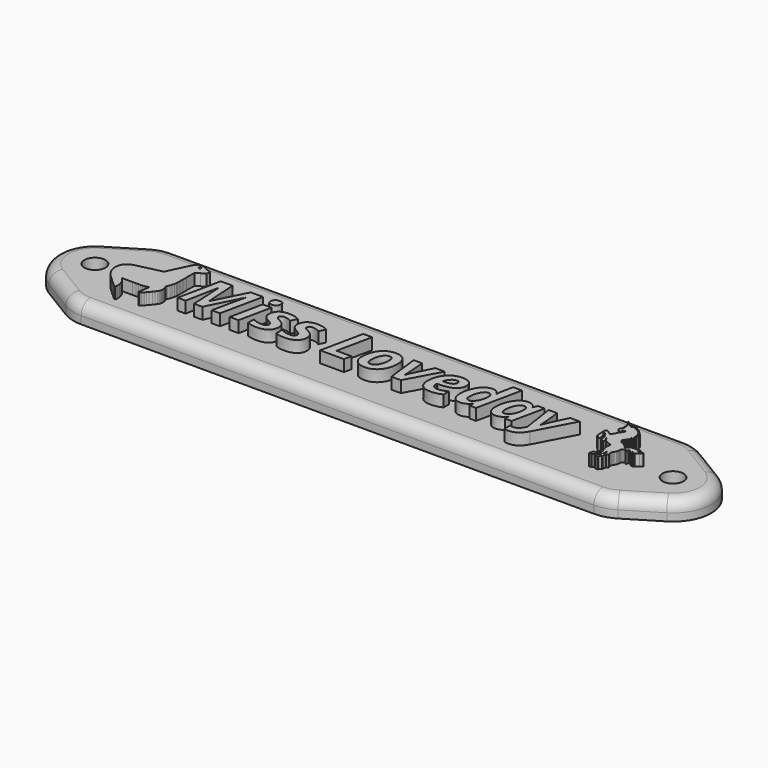
from build123d import *

# Parameters (mm, degrees)
F0_W         = 140
F0_H         = 30.4531101137
F1_DEPTH     = 5
F2_R         = 10
F3_R         = 10
F4_TEXT_SIZE = 15.6755168022
F5_DEPTH     = 3
F7_D         = 5.5
F8_R         = 0.282704
F9_DEPTH     = 3
F11_DEPTH    = 3
F12_R        = 3


# Not quite as in the source:
# - Text() gives the source's letters only with a copy of the font that has no kerning and outlines rounded to 1/6400 em; it was checked with that copy


with BuildPart() as f1:
    # F0 (on Top) → F1 (new body)
    with BuildSketch(Plane.XY):
        Rectangle(F0_W, F0_H)
        Polygon((-95, 0), (-70, -15.2265550569), (-70, 15.2265550569), align=None)
        Polygon((70, 15.2265550569), (70, -15.2265550569), (95, 0), align=None)
    extrude(amount=F1_DEPTH)

    # F2
    f2_edges = [f1.edges().sort_by_distance(p)[0] for p in [
        (-95, 0, 2.5),
        (95, 0, 2.5),
    ]]
    fillet(f2_edges, radius=F2_R)

    # F3
    f3_edges = [f1.edges().sort_by_distance(p)[0] for p in [
        (70, -15.226555, 2.5),
        (-70, -15.226555, 2.5),
        (-70, 15.226555, 2.5),
        (70, 15.226555, 2.5),
    ]]
    fillet(f3_edges, radius=F3_R)

    # F4 (on face) → F5 (join)
    with BuildSketch(Plane.XY.offset(5)):
        with Locations((-50, -5.6431860488)):
            Text('Miss Loveday', F4_TEXT_SIZE, font='Open Sans', font_style=FontStyle.BOLDITALIC, text_align=(TextAlign.LEFT, TextAlign.BOTTOM))
    extrude(amount=F5_DEPTH)

    # F7 (through all)
    with Locations(Plane.XY.offset(5)):
        with Locations((75.7757134551, 0), (-75.7757134551, 0)):
            Hole(F7_D / 2)

    # F8 (on face) → F9 (join)
    with BuildSketch(Plane.XY.offset(5)):
        Polygon((-65.1555724097, -7.7435036488), (-64.4543324097, -8.3903836488), (-63.8004924097, -8.9847836488), (-63.3014124097, -9.4225036488), (-62.9708524097, -9.6913836488), (-62.8232924097, -9.7795036488), (-62.7180524097, -9.7196236488), (-62.6414524097, -9.5731036488), (-62.5945724097, -9.3429036488), (-62.5787324097, -9.0325436488), (-62.6422924097, -8.3105436488), (-62.8250124097, -7.6104636488), (-63.1164524097, -6.9641836488), (-63.5049724097, -6.4027836488), (-63.8716924097, -5.9724636488), (-61.1974124097, -5.9719836488), (-60.2803324097, -5.9702636488), (-59.5541724097, -5.9641836488), (-58.9880124097, -5.9516236488), (-58.5498524097, -5.9301036488), (-58.2078524097, -5.8975436488), (-57.9307324097, -5.8519836488), (-57.6867724097, -5.7909836488), (-57.4439324097, -5.7126636488), (-57.2961724097, -5.6636236488), (-57.1685724097, -5.6267036488), (-57.0750124097, -5.6049836488), (-57.0287724097, -5.6023836488), (-57.0309724097, -5.7204636488), (-57.0682924097, -6.0279836488), (-57.1347324097, -6.4782636488), (-57.2236924097, -7.0245036488), (-57.3161324097, -7.5752636488), (-57.3918524097, -8.0383836488), (-57.4430524097, -8.3649836488), (-57.4619724097, -8.5067036488), (-57.4274524097, -8.6149836488), (-57.3402124097, -8.7239436488), (-57.2267324097, -8.8077036488), (-57.1134524097, -8.8413436488), (-57.0650524097, -8.8237836488), (-56.9908524097, -8.7684236488), (-56.8868924097, -8.6705436488), (-56.7486124097, -8.5251836488), (-56.5720124097, -8.3274636488), (-56.3524124097, -8.0729036488), (-56.0854524097, -7.7567036488), (-55.7666924097, -7.3743436488), (-55.2898924097, -6.7946636488), (-54.9224524097, -6.3341836488), (-54.6503324097, -5.9682636488), (-54.4593324097, -5.6722636488), (-54.3354524097, -5.4220636488), (-54.2646924097, -5.1931036488), (-54.2330124097, -4.9611036488), (-54.2260524097, -4.7016236488), (-54.2434524097, -4.3704636488), (-54.2978924097, -4.0781036488), (-54.3979324097, -3.7933836488), (-54.5517724097, -3.4861036488), (-54.5795724097, -3.4335436488), (-54.5974124097, -3.3871036488), (-54.6041324097, -3.3402636488), (-54.5982124097, -3.2871036488), (-54.5782924097, -3.2206636488), (-54.5431324097, -3.1349436488), (-54.4912924097, -3.0236236488), (-54.4211724097, -2.8803836488), (-54.2238924097, -2.4136236488), (-54.0481324097, -1.8749836488), (-53.9085724097, -1.3157036488), (-53.8202124097, -0.7879436488), (-53.7970124097, -0.3858236488), (-53.7783324097, 0.3344563512), (-53.7664524097, 1.2940563512), (-53.7618924097, 2.4142963512), (-53.7618924097, 5.1182563512), (-52.7145724097, 5.7410563512), (-51.6670524097, 6.3638563512), (-51.5784924097, 6.6506563512), (-51.4904124097, 6.9626563512), (-51.4482924097, 7.1830563512), (-51.4504524097, 7.3322563512), (-51.4949324097, 7.4282563512), (-51.5828524097, 7.4782563512), (-51.7638524097, 7.5458563512), (-52.0116924097, 7.6226563512), (-52.2998524097, 7.6994563512), (-52.8927324097, 7.8718563512), (-53.1930524097, 8.0278563512), (-53.5574524097, 8.2766563512), (-53.9817324097, 8.4458563512), (-54.4176924097, 8.5214563512), (-54.8158924097, 8.4890563512), (-55.1251724097, 8.3802563512), (-55.4367724097, 8.2134563512), (-55.7232124097, 8.0058563512), (-55.9565724097, 7.7746563512), (-56.0316124097, 7.6666563512), (-56.1398924097, 7.4810563512), (-56.2824924097, 7.2146563512), (-56.4614924097, 6.8650563512), (-56.6783324097, 6.4282563512), (-56.9344124097, 5.9018563512), (-57.2314924097, 5.2826563512), (-57.5708924097, 4.5666563512), (-58.9584924097, 1.6295363512), (-62.2777324097, 0.8522163512), (-62.9506924097, 0.6942163512), (-63.5902124097, 0.5427763512), (-64.1817724097, 0.4017363512), (-64.7100124097, 0.2745763512), (-65.1604924097, 0.1651763512), (-65.5184124097, 0.0766163512), (-65.7686124097, 0.0130563512), (-65.8964524097, -0.0225436488), (-66.6711724097, -0.3808236488), (-67.2807324097, -0.8839036488), (-67.7200124097, -1.5086636488), (-67.9834524097, -2.2315436488), (-68.0661324097, -3.0292636488), (-67.9624124097, -3.8786636488), (-67.6670524097, -4.7565036488), (-67.1748524097, -5.6395036488), (-67.0285724097, -5.8496236488), (-66.8744924097, -6.0496636488), (-66.6891724097, -6.2636636488), (-66.4484924097, -6.5158236488), (-66.1286124097, -6.8305036488), (-65.7056924097, -7.2315436488), align=None)
        with Locations((-54.2613854097, 7.5656233512)):
            Circle(F8_R, mode=Mode.SUBTRACT)
    extrude(amount=F9_DEPTH)

    # F10 (on face) → F11 (join)
    with BuildSketch(Plane.XY.offset(5)):
        Polygon((59.2275306848, -6.5195911563), (59.1261026848, -6.8110191563), (59.1469596848, -6.8247341563), (59.1698166848, -6.8364481563), (59.2069596848, -6.8507341563), (59.2478166848, -6.8615911563), (59.3066736848, -6.8713051563), (59.6141026848, -6.8735911563), (59.9246736848, -6.8724481563), (59.9561026848, -6.8524481563), (59.9843876848, -6.8293051563), (60.0101026848, -6.8033051563), (60.0406736848, -6.7650191563), (60.0743876848, -6.7127341563), (60.2169596848, -6.4598771563), (60.2481026848, -6.4221621563), (60.2652446848, -6.4047341563), (60.2929596848, -6.3813051563), (60.3095306848, -6.3984481563), (60.3252446848, -6.4113051563), (60.3395306848, -6.4204481563), (60.3466736848, -6.4235911563), (60.3532446848, -6.4258771563), (60.3598166848, -6.4273051563), (60.3661026848, -6.4281621563), (60.3723876848, -6.4281621563), (60.3783876848, -6.4275911563), (60.3841026848, -6.4264481563), (60.3898166848, -6.4244481563), (60.4009596848, -6.4195911563), (60.4115306848, -6.4127341563), (60.4266736848, -6.4001621563), (60.4818166848, -6.3495911563), (60.4923876848, -6.3427341563), (60.5035306848, -6.3378771563), (60.5092446848, -6.3361621563), (60.5149596848, -6.3347341563), (60.5209596848, -6.3341621563), (60.5272446848, -6.3341621563), (60.5335306848, -6.3350191563), (60.5401026848, -6.3364481563), (60.5466736848, -6.3387341563), (60.5535306848, -6.3418771563), (60.5681026848, -6.3510191563), (60.5835306848, -6.3638771563), (60.6001026848, -6.3813051563), (60.6026736848, -6.3321621563), (60.6095306848, -6.2873051563), (60.6201026848, -6.2464481563), (60.6386736848, -6.1961621563), (60.6672446848, -6.1387341563), (60.7521026848, -5.9827341563), (60.7709596848, -5.9327341563), (60.7815306848, -5.8918771563), (60.7886736848, -5.8473051563), (60.7915306848, -5.7984481563), (60.7903876848, -5.7633051563), (60.7843876848, -5.7055911563), (60.8186736848, -5.6941621563), (60.8503876848, -5.6793051563), (60.8803876848, -5.6610191563), (60.9083876848, -5.6401621563), (60.9438166848, -5.6084481563), (61.0766736848, -5.4427341563), (61.2143876848, -5.2755911563), (61.2192446848, -5.2715911563), (61.2246736848, -5.2678771563), (61.2338166848, -5.2627341563), (61.2478166848, -5.2570191563), (61.2715306848, -5.2501621563), (61.3755306848, -5.2258771563), (61.3881026848, -5.2207341563), (61.3938166848, -5.2175911563), (61.3986736848, -5.2141621563), (61.4606736848, -5.1553051563), (61.5215306848, -5.0913051563), (61.5726736848, -5.0298771563), (61.6121026848, -4.9693051563), (61.6409596848, -4.9095911563), (61.6603876848, -4.8501621563), (61.6721026848, -4.7913051563), (61.6769596848, -4.7324481563), (61.6752446848, -4.6538771563), (61.6269596848, -4.1904481563), (61.6321026848, -4.1201621563), (61.6443876848, -4.0473051563), (61.7003876848, -4.1458771563), (61.7478166848, -4.2533051563), (61.7858166848, -4.3701621563), (61.8138166848, -4.4970191563), (61.8309596848, -4.6344481563), (61.8366736848, -4.7835911563), (61.8286736848, -4.9684481563), (61.7061026848, -5.0818771563), (61.5386736848, -5.2684481563), (61.2452446848, -5.6430191563), (60.9072446848, -6.0127341563), (60.9198166848, -6.0990191563), (60.9229596848, -6.1758771563), (60.9183876848, -6.2447341563), (60.9072446848, -6.3075911563), (60.8869596848, -6.3793051563), (60.7981026848, -6.6404481563), (60.7875306848, -6.7035911563), (60.7838166848, -6.7553051563), (60.7843876848, -6.8110191563), (60.8012446848, -6.8238771563), (60.8195306848, -6.8350191563), (60.8395306848, -6.8444481563), (60.8721026848, -6.8561621563), (60.9078166848, -6.8647341563), (60.9592446848, -6.8724481563), (61.2086736848, -6.8733051563), (61.4601026848, -6.8724481563), (61.4638166848, -6.8615911563), (61.4683876848, -6.8515911563), (61.4726736848, -6.8444481563), (61.4772446848, -6.8381621563), (61.4826736848, -6.8324481563), (61.4886736848, -6.8273051563), (61.4949596848, -6.8227341563), (61.5021026848, -6.8190191563), (61.5101026848, -6.8155911563), (61.5183876848, -6.8130191563), (61.5306736848, -6.8104481563), (61.5441026848, -6.8090191563), (61.5623876848, -6.8090191563), (61.5829596848, -6.8110191563), (61.5955306848, -6.7573051563), (61.6135306848, -6.7093051563), (61.6366736848, -6.6658771563), (61.6635306848, -6.6264481563), (61.7043876848, -6.5787341563), (61.9272446848, -6.3595911563), (61.9543876848, -6.3201621563), (61.9772446848, -6.2767341563), (61.9955306848, -6.2287341563), (62.0043876848, -6.1935911563), (62.0129596848, -6.1355911563), (62.1969596848, -6.1355911563), (62.1995306848, -5.9915911563), (62.2275306848, -5.7481621563), (62.2661026848, -5.4318771563), (62.2689596848, -5.3093051563), (62.2583876848, -5.1527341563), (62.2926736848, -5.1133051563), (62.3401026848, -5.0684481563), (62.4126736848, -5.0121621563), (62.6481026848, -4.8421621563), (62.6943876848, -4.7964481563), (62.7198166848, -4.7664481563), (62.7498166848, -4.7230191563), (62.7483876848, -4.6904481563), (62.7435306848, -4.6584481563), (62.7332446848, -4.6155911563), (62.7146736848, -4.5621621563), (62.5821026848, -4.2530191563), (62.5732446848, -4.2178771563), (62.5655306848, -4.1701621563), (62.5589596848, -4.0493051563), (62.5638166848, -3.9367341563), (62.5786736848, -3.8324481563), (62.6021026848, -3.7353051563), (62.6412446848, -3.6230191563), (62.6986736848, -3.5010191563), (62.8169596848, -3.3067341563), (62.9341026848, -3.1258771563), (63.1298166848, -2.7533051563), (63.2312446848, -2.5078771563), (63.2715306848, -2.3861621563), (63.3026736848, -2.2661621563), (63.3198166848, -2.1653051563), (63.3315306848, -2.0133051563), (63.3415306848, -1.6253051563), (63.3492446848, -1.5790191563), (63.3543876848, -1.5581621563), (63.3641026848, -1.5290191563), (63.3886736848, -1.4750191563), (63.4286736848, -1.4064481563), (63.4758166848, -1.3413051563), (63.5432446848, -1.2653051563), (63.6181026848, -1.1953051563), (63.7155306848, -1.1195911563), (63.8346736848, -1.0427341563), (63.9715306848, -0.9701621563), (64.1009596848, -0.9150191563), (64.1463876848, -0.9321621563), (64.1872446848, -0.9541621563), (64.2238166848, -0.9798771563), (64.2569596848, -1.0095911563), (64.2869596848, -1.0424481563), (64.3223876848, -1.0904481563), (64.3609596848, -1.1561621563), (64.4263876848, -1.2995911563), (64.4758166848, -1.4173051563), (64.5309596848, -1.5290191563), (64.5538166848, -1.4598771563), (64.5803876848, -1.3390191563), (64.6495306848, -0.9473051563), (64.6721026848, -0.8778771563), (64.6889596848, -0.8393051563), (64.7152446848, -0.7921621563), (65.1452446848, -0.7921621563), (65.2666736848, -0.9138771563), (65.6092446848, -1.2344481563), (65.6501026848, -1.2821621563), (65.6978166848, -1.3447341563), (65.7478166848, -1.3498771563), (66.1275306848, -1.4144481563), (66.1883876848, -1.4138771563), (66.2306736848, -1.4081621563), (66.2569596848, -1.4013051563), (66.2812446848, -1.3918771563), (66.3035306848, -1.3795911563), (66.3238166848, -1.3644481563), (66.3415306848, -1.3458771563), (66.3563876848, -1.3235911563), (66.3629596848, -1.3113051563), (66.3735306848, -1.2833051563), (66.2275306848, -1.2821621563), (66.1441026848, -1.2733051563), (66.0823876848, -1.2613051563), (66.0261026848, -1.2438771563), (65.9875306848, -1.2273051563), (65.9523876848, -1.2070191563), (65.9309596848, -1.1915911563), (65.9112446848, -1.1744481563), (65.8932446848, -1.1555911563), (65.8772446848, -1.1350191563), (65.8629596848, -1.1124481563), (65.8506736848, -1.0878771563), (65.8403876848, -1.0613051563), (65.8321026848, -1.0327341563), (65.8238166848, -0.9855911563), (65.8212446848, -0.9513051563), (65.8206736848, -0.9150191563), (65.8769596848, -0.9215911563), (65.9286736848, -0.9324481563), (65.9921026848, -0.9524481563), (66.0501026848, -0.9781621563), (66.1301026848, -1.0233051563), (66.3486736848, -1.1595911563), (66.4066736848, -1.1853051563), (66.4695306848, -1.2058771563), (66.5035306848, -1.2135911563), (66.5578166848, -1.2218771563), (66.5652446848, -1.2207341563), (66.5718166848, -1.2190191563), (66.5781026848, -1.2164481563), (66.5838166848, -1.2135911563), (66.5892446848, -1.2104481563), (66.5941026848, -1.2064481563), (66.5983876848, -1.2024481563), (66.6023876848, -1.1978771563), (66.6092446848, -1.1875911563), (66.6149596848, -1.1758771563), (66.6195306848, -1.1633051563), (66.6246736848, -1.1427341563), (66.6441026848, -1.0330191563), (66.6486736848, -1.0204481563), (66.6543876848, -1.0090191563), (66.6615306848, -0.9987341563), (66.6655306848, -0.9944481563), (66.6698166848, -0.9901621563), (66.6746736848, -0.9864481563), (66.6801026848, -0.9833051563), (66.6861026848, -0.9804481563), (66.6923876848, -0.9781621563), (66.6992446848, -0.9764481563), (66.7143876848, -0.9744481563), (66.7229596848, -0.9744481563), (66.7421026848, -0.9764481563), (67.4178166848, -0.5464481563), (67.8358166848, -0.3101621563), (67.8895306848, -0.2658771563), (67.9255306848, -0.2293051563), (67.9578166848, -0.1895911563), (67.9849596848, -0.1464481563), (68.0069596848, -0.0995911563), (68.0181026848, -0.0661621563), (68.0266736848, -0.0310191563), (68.0318166848, 0.0064088437), (67.9761026848, 0.0318378437), (67.9172446848, 0.0512658437), (67.8558166848, 0.0652658437), (67.7595306848, 0.0766948437), (67.6249596848, 0.0784088437), (67.3783876848, 0.0549808437), (66.8869596848, -0.0018771563), (66.7578166848, 0.0009808437), (66.6669596848, 0.0138378437), (66.6098166848, 0.0289808437), (66.5555306848, 0.0492658437), (66.5046736848, 0.0761228437), (66.4803876848, 0.0921228437), (66.4349596848, 0.1292658437), (66.4572446848, 0.1621228437), (66.4823876848, 0.1924088437), (66.5192446848, 0.2292658437), (66.5701026848, 0.2704088437), (66.8421026848, 0.4592658437), (66.8789596848, 0.4958378437), (66.9041026848, 0.5261228437), (66.9263876848, 0.5592658437), (66.6349596848, 0.5212658437), (66.2906736848, 0.5109808437), (64.8941026848, 0.5749808437), (64.7203876848, 0.5506948437), (64.5975306848, 0.5192658437), (64.5192446848, 0.4909808437), (64.4081026848, 0.4364088437), (64.2852446848, 0.3569808437), (64.1538166848, 0.2541228437), (63.5326736848, -0.3198771563), (63.4635306848, -0.3661621563), (63.3641026848, -0.4235911563), (63.3063876848, -0.2847341563), (63.2363876848, -0.1581621563), (63.1552446848, -0.0427341563), (63.0638166848, 0.0624088437), (62.9103876848, 0.2038378437), (62.7406736848, 0.3286948437), (62.4321026848, 0.5115518437), (61.5375306848, 0.9929808437), (61.3669596848, 1.1172658437), (61.2123876848, 1.2575518437), (61.1203876848, 1.3618378437), (61.0381026848, 1.4761228437), (60.9669596848, 1.6015518437), (60.9083876848, 1.7395518437), (60.8841026848, 1.8132658437), (60.8458166848, 1.9718378437), (60.8883876848, 2.0469808437), (60.9089596848, 2.0755518437), (60.9275306848, 2.0966948437), (60.9426736848, 2.1106948437), (60.9595306848, 2.1235518437), (60.9778166848, 2.1346948437), (60.9978166848, 2.1441228437), (61.0198166848, 2.1518378437), (61.0438166848, 2.1569808437), (61.0701026848, 2.1601228437), (61.0989596848, 2.1609808437), (61.1195306848, 2.1598378437), (61.1529596848, 2.1561228437), (61.1612446848, 2.1744088437), (61.1666736848, 2.1924088437), (61.1701026848, 2.2104088437), (61.1712446848, 2.2281228437), (61.1703876848, 2.2455518437), (61.1663876848, 2.2712658437), (61.1598166848, 2.2961228437), (61.1478166848, 2.3272658437), (61.1086736848, 2.4166948437), (61.1066736848, 2.4261228437), (61.1063876848, 2.4306948437), (61.1063876848, 2.4346948437), (61.1069596848, 2.4386948437), (61.1081026848, 2.4424088437), (61.1095306848, 2.4458378437), (61.1118166848, 2.4486948437), (61.1143876848, 2.4515518437), (61.1178166848, 2.4541228437), (61.1218166848, 2.4564088437), (61.1266736848, 2.4584088437), (61.1321026848, 2.4601228437), (61.1381026848, 2.4612658437), (61.1529596848, 2.4632658437), (61.1729596848, 2.4646948437), (61.1909596848, 2.4641228437), (61.2072446848, 2.4621228437), (61.2223876848, 2.4589808437), (61.2409596848, 2.4526948437), (61.2621026848, 2.4432658437), (61.3232446848, 2.4124088437), (61.3418166848, 2.4064088437), (61.3572446848, 2.4032658437), (61.3738166848, 2.4015518437), (61.3858166848, 2.4012658437), (61.3986736848, 2.4018378437), (61.4681026848, 2.6566948437), (61.4861026848, 2.6975518437), (61.5021026848, 2.7255518437), (61.5206736848, 2.7512658437), (61.5346736848, 2.7666948437), (61.5501026848, 2.7809808437), (61.5669596848, 2.7935518437), (61.5855306848, 2.8046948437), (61.6055306848, 2.8138378437), (61.6275306848, 2.8212658437), (61.6515306848, 2.8269808437), (61.6775306848, 2.8304088437), (61.7058166848, 2.8315518437), (61.6746736848, 2.9669808437), (61.6735306848, 2.9815518437), (61.6741026848, 2.9958378437), (61.6835306848, 3.0461228437), (61.7058166848, 3.1386948437), (61.7255306848, 3.1401228437), (61.7438166848, 3.1398378437), (61.7601026848, 3.1378378437), (61.7752446848, 3.1344088437), (61.7935306848, 3.1284088437), (61.8146736848, 3.1186948437), (61.8761026848, 3.0881228437), (61.8946736848, 3.0821228437), (61.9098166848, 3.0789808437), (61.9266736848, 3.0769808437), (61.9386736848, 3.0766948437), (61.9515306848, 3.0772658437), (61.9629596848, 3.1369808437), (61.9675306848, 3.1935518437), (61.9658166848, 3.2475518437), (61.9592446848, 3.2986948437), (61.9446736848, 3.3635518437), (61.9092446848, 3.4681228437), (61.8615306848, 3.6032658437), (61.8529596848, 3.6415518437), (61.8489596848, 3.6789808437), (61.8492446848, 3.7038378437), (61.8523876848, 3.7284088437), (61.8586736848, 3.7529808437), (61.8683876848, 3.7775518437), (61.8746736848, 3.7898378437), (61.8901026848, 3.8144088437), (61.9301026848, 3.8101228437), (61.9761026848, 3.8009808437), (62.0266736848, 3.7852658437), (62.2338166848, 3.7049808437), (62.2703876848, 3.6972658437), (62.3198166848, 3.6915518437), (62.3098166848, 3.8041228437), (62.2903876848, 3.9075518437), (62.2572446848, 4.0218378437), (62.1938166848, 4.1795518437), (62.1001026848, 4.3806948437), (62.0129596848, 4.6126948437), (62.0946736848, 4.6686948437), (62.1215306848, 4.6921228437), (62.1361026848, 4.7084088437), (62.1435306848, 4.7192658437), (62.1489596848, 4.7298378437), (62.1529596848, 4.7404088437), (62.1549596848, 4.7512658437), (62.1558166848, 4.7624088437), (62.1549596848, 4.7741228437), (62.1526736848, 4.7861228437), (62.1472446848, 4.8058378437), (62.1175306848, 4.8784088437), (62.0741026848, 4.9812658437), (62.1566736848, 5.0106948437), (62.2218166848, 5.0412658437), (62.2715306848, 5.0715518437), (62.3075306848, 5.0992658437), (62.3401026848, 5.1306948437), (62.3621026848, 5.1566948437), (62.3815306848, 5.1849808437), (62.3986736848, 5.2158378437), (62.4132446848, 5.2489808437), (62.4252446848, 5.2852658437), (62.4341026848, 5.3241228437), (62.4401026848, 5.3661228437), (62.4426736848, 5.4112658437), (62.1975306848, 5.4118378437), (62.1318166848, 5.4195518437), (62.0912446848, 5.4284088437), (62.0632446848, 5.4369808437), (62.0372446848, 5.4481228437), (62.0138166848, 5.4612658437), (61.9995306848, 5.4715518437), (61.9866736848, 5.4832658437), (61.9746736848, 5.4961228437), (61.9643876848, 5.5101228437), (61.9598166848, 5.5178378437), (61.9515306848, 5.5341228437), (61.9652446848, 5.7164088437), (61.9761026848, 5.8249808437), (61.9752446848, 5.8698378437), (61.9675306848, 5.9355518437), (61.9515306848, 6.0255518437), (62.0106736848, 6.0324088437), (62.0532446848, 6.0415518437), (62.0863876848, 6.0524088437), (62.1118166848, 6.0638378437), (62.1306736848, 6.0746948437), (62.1478166848, 6.0869808437), (62.1632446848, 6.1009808437), (62.1738166848, 6.1124088437), (62.1835306848, 6.1249808437), (62.1892446848, 6.1338378437), (62.1969596848, 6.1484088437), (62.1403876848, 6.1749808437), (62.0638166848, 6.2026948437), (61.9143876848, 6.2415518437), (61.5581026848, 6.3238378437), (61.4818166848, 6.3518378437), (61.4386736848, 6.3715518437), (61.3986736848, 6.3938378437), (61.3915306848, 6.4178378437), (61.3875306848, 6.4412658437), (61.3861026848, 6.4646948437), (61.3866736848, 6.4878378437), (61.3915306848, 6.5221228437), (61.4029596848, 6.5666948437), (61.4641026848, 6.7395518437), (61.4669596848, 6.7578378437), (61.4683876848, 6.7755518437), (61.4672446848, 6.7929808437), (61.4638166848, 6.8098378437), (61.4575306848, 6.8261228437), (61.4481026848, 6.8418378437), (61.4355306848, 6.8566948437), (61.4189596848, 6.8712658437), (61.3986736848, 6.8852658437), (61.3749596848, 6.8666948437), (61.2441026848, 6.7486948437), (61.2258166848, 6.7375518437), (61.2075306848, 6.7289808437), (61.1949596848, 6.7249808437), (61.1826736848, 6.7224088437), (61.1698166848, 6.7218378437), (61.1572446848, 6.7229808437), (61.1443876848, 6.7264088437), (61.1312446848, 6.7315518437), (61.1183876848, 6.7395518437), (61.1049596848, 6.7495518437), (61.0915306848, 6.7624088437), (61.0881026848, 6.8326948437), (61.0786736848, 6.8969808437), (61.0586736848, 6.9801228437), (60.9815306848, 7.2421228437), (60.9721026848, 7.3064088437), (60.9686736848, 7.3766948437), (60.9463876848, 7.3815518437), (60.9269596848, 7.3838378437), (60.9101026848, 7.3838378437), (60.8955306848, 7.3812658437), (60.8889596848, 7.3789808437), (60.8829596848, 7.3764088437), (60.8772446848, 7.3735518437), (60.8721026848, 7.3701228437), (60.8675306848, 7.3661228437), (60.8592446848, 7.3572658437), (60.8521026848, 7.3469808437), (60.8461026848, 7.3358378437), (60.8386736848, 7.3175518437), (60.8129596848, 7.2401228437), (60.8069596848, 7.2289808437), (60.7998166848, 7.2186948437), (60.7915306848, 7.2098378437), (60.7869596848, 7.2058378437), (60.7818166848, 7.2024088437), (60.7763876848, 7.1992658437), (60.7703876848, 7.1966948437), (60.7638166848, 7.1946948437), (60.7569596848, 7.1929808437), (60.7412446848, 7.1915518437), (60.7229596848, 7.1924088437), (60.4975306848, 7.1929808437), (60.4635306848, 7.1984088437), (60.4403876848, 7.2044088437), (60.4192446848, 7.2126948437), (60.4063876848, 7.2195518437), (60.3946736848, 7.2278378437), (60.3843876848, 7.2369808437), (60.3755306848, 7.2478378437), (60.3681026848, 7.2601228437), (60.3621026848, 7.2735518437), (60.3578166848, 7.2889808437), (60.3563876848, 7.2972658437), (60.3543876848, 7.3152658437), (60.3458166848, 7.3412658437), (60.3412446848, 7.3629808437), (60.3401026848, 7.3812658437), (60.3409596848, 7.3889808437), (60.3423876848, 7.3961228437), (60.3446736848, 7.4024088437), (60.3478166848, 7.4081228437), (60.3512446848, 7.4129808437), (60.3555306848, 7.4172658437), (60.3603876848, 7.4212658437), (60.3658166848, 7.4244088437), (60.3715306848, 7.4272658437), (60.3843876848, 7.4315518437), (60.3986736848, 7.4344088437), (60.4301026848, 7.4372658437), (60.4943876848, 7.4418378437), (60.5086736848, 7.4446948437), (60.5218166848, 7.4489808437), (60.5275306848, 7.4518378437), (60.5329596848, 7.4549808437), (60.5378166848, 7.4586948437), (60.5421026848, 7.4629808437), (60.5455306848, 7.4681228437), (60.5486736848, 7.4735518437), (60.5509596848, 7.4801228437), (60.5523876848, 7.4869808437), (60.5532446848, 7.4949808437), (60.5532446848, 7.5035518437), (60.5503876848, 7.5235518437), (60.5475306848, 7.5349808437), (60.5386736848, 7.5609808437), (60.5335306848, 7.5704088437), (60.5272446848, 7.5789808437), (60.5201026848, 7.5864088437), (60.5121026848, 7.5929808437), (60.5029596848, 7.5989808437), (60.4932446848, 7.6038378437), (60.4718166848, 7.6118378437), (60.4475306848, 7.6169808437), (60.4072446848, 7.6209808437), (60.3332446848, 7.6206948437), (60.1669596848, 7.6166948437), (60.1278166848, 7.6215518437), (60.1043876848, 7.6275518437), (60.0835306848, 7.6364088437), (60.0743876848, 7.6418378437), (60.0658166848, 7.6481228437), (60.0583876848, 7.6552658437), (60.0518166848, 7.6635518437), (60.0461026848, 7.6724088437), (60.0415306848, 7.6826948437), (60.0378166848, 7.6938378437), (60.0355306848, 7.7061228437), (60.0341026848, 7.7195518437), (60.0355306848, 7.7504088437), (60.0381026848, 7.7678378437), (60.0475306848, 7.8066948437), (60.0215306848, 7.8081228437), (59.9981026848, 7.8069808437), (59.9769596848, 7.8032658437), (59.9581026848, 7.7978378437), (59.9409596848, 7.7901228437), (59.9255306848, 7.7809808437), (59.9115306848, 7.7706948437), (59.8923876848, 7.7526948437), (59.8641026848, 7.7195518437), (59.8195306848, 7.6661228437), (59.8001026848, 7.6484088437), (59.7861026848, 7.6381228437), (59.7703876848, 7.6292658437), (59.7529596848, 7.6218378437), (59.7338166848, 7.6164088437), (59.7126736848, 7.6132658437), (59.6889596848, 7.6124088437), (59.6623876848, 7.6141228437), (59.6175306848, 7.6224088437), (59.6141026848, 7.6372658437), (59.6092446848, 7.6509808437), (59.6032446848, 7.6635518437), (59.5963876848, 7.6749808437), (59.5858166848, 7.6889808437), (59.5681026848, 7.7081228437), (59.5223876848, 7.7544088437), (59.5118166848, 7.7684088437), (59.5049596848, 7.7801228437), (59.4992446848, 7.7926948437), (59.4946736848, 7.8066948437), (59.4966736848, 7.8412658437), (59.5023876848, 7.8724088437), (59.5115306848, 7.9001228437), (59.5232446848, 7.9252658437), (59.5372446848, 7.9481228437), (59.5583876848, 7.9764088437), (59.6412446848, 8.0775518437), (59.6546736848, 8.1009808437), (59.6658166848, 8.1269808437), (59.6738166848, 8.1555518437), (59.6786736848, 8.1875518437), (59.6798166848, 8.2109808437), (59.6789596848, 8.2364088437), (59.5952446848, 8.2169808437), (59.5186736848, 8.1904088437), (59.4481026848, 8.1578378437), (59.3612446848, 8.1069808437), (59.2621026848, 8.0344088437), (58.9206736848, 7.7566948437), (58.8338166848, 7.7058378437), (58.7632446848, 7.6732658437), (58.6866736848, 7.6466948437), (58.6315306848, 7.6329808437), (58.5732446848, 7.6224088437), (58.5746736848, 7.8961228437), (58.5809596848, 7.9389808437), (58.5883876848, 7.9709808437), (58.5961026848, 7.9926948437), (58.6052446848, 8.0129808437), (58.6163876848, 8.0312658437), (58.6252446848, 8.0421228437), (58.6346736848, 8.0521228437), (58.6061026848, 8.0501228437), (58.5789596848, 8.0449808437), (58.5535306848, 8.0372658437), (58.5295306848, 8.0266948437), (58.5069596848, 8.0141228437), (58.4755306848, 7.9918378437), (58.4466736848, 7.9664088437), (58.4035306848, 7.9204088437), (58.3106736848, 7.8118378437), (58.2978166848, 7.8006948437), (58.2849596848, 7.7918378437), (58.2721026848, 7.7855518437), (58.2658166848, 7.7835518437), (58.2592446848, 7.7824088437), (58.2526736848, 7.7821228437), (58.2461026848, 7.7826948437), (58.2395306848, 7.7841228437), (58.2326736848, 7.7864088437), (58.2258166848, 7.7898378437), (58.2189596848, 7.7944088437), (58.2121026848, 7.7998378437), (58.2049596848, 7.8066948437), (58.1581026848, 7.8489808437), (58.1015306848, 7.8906948437), (58.0046736848, 7.9486948437), (57.8758166848, 8.0221228437), (57.8581026848, 8.0346948437), (57.8363876848, 8.0521228437), (57.6346736848, 8.2529808437), (57.2026736848, 8.7398378437), (56.8535306848, 9.0964088437), (56.8435306848, 9.1029808437), (56.8046736848, 9.1244088437), (56.7452446848, 9.1506948437), (56.7009596848, 9.1655518437), (56.6766736848, 9.1712658437), (56.6595306848, 9.1735518437), (56.6441026848, 9.1738378437), (56.6346736848, 9.1729808437), (56.6263876848, 9.1709808437), (56.6226736848, 9.1695518437), (56.6189596848, 9.1678378437), (56.6158166848, 9.1658378437), (56.6129596848, 9.1635518437), (56.6103876848, 9.1606948437), (56.6081026848, 9.1578378437), (57.2415306848, 8.2866948437), (57.8363876848, 7.3766948437), (57.8226736848, 7.3458378437), (57.8069596848, 7.3175518437), (57.7886736848, 7.2915518437), (57.7718166848, 7.2718378437), (57.7532446848, 7.2535518437), (57.7286736848, 7.2338378437), (57.7018166848, 7.2161228437), (57.6778166848, 7.2035518437), (57.6521026848, 7.1924088437), (57.6718166848, 7.1672658437), (57.6863876848, 7.1426948437), (57.6961026848, 7.1192658437), (57.7012446848, 7.0961228437), (57.7023876848, 7.0738378437), (57.7001026848, 7.0521228437), (57.6946736848, 7.0309808437), (57.6866736848, 7.0104088437), (57.6709596848, 6.9804088437), (57.6446736848, 6.9418378437), (57.5721026848, 6.8421228437), (57.5629596848, 6.8244088437), (57.5561026848, 6.8069808437), (57.5521026848, 6.7895518437), (57.5512446848, 6.7806948437), (57.5515306848, 6.7721228437), (57.5523876848, 6.7632658437), (57.5543876848, 6.7544088437), (57.5575306848, 6.7455518437), (57.5618166848, 6.7366948437), (57.5669596848, 6.7278378437), (57.5735306848, 6.7189808437), (57.5906736848, 6.7009808437), (57.5923876848, 6.7092658437), (57.5946736848, 6.7166948437), (57.5975306848, 6.7235518437), (57.6012446848, 6.7298378437), (57.6055306848, 6.7355518437), (57.6103876848, 6.7404088437), (57.6155306848, 6.7449808437), (57.6215306848, 6.7486948437), (57.6281026848, 6.7521228437), (57.6383876848, 6.7564088437), (57.6501026848, 6.7595518437), (57.6666736848, 6.7626948437), (57.6938166848, 6.7649808437), (57.7335306848, 6.7646948437), (57.7749596848, 6.7624088437), (57.7326736848, 6.6906948437), (57.7215306848, 6.6664088437), (57.7175306848, 6.6535518437), (57.7158166848, 6.6435518437), (57.7158166848, 6.6392658437), (57.7163876848, 6.6355518437), (57.7175306848, 6.6324088437), (57.7189596848, 6.6298378437), (57.7209596848, 6.6275518437), (57.7235306848, 6.6255518437), (57.7263876848, 6.6241228437), (57.7298166848, 6.6229808437), (57.7335306848, 6.6221228437), (57.7418166848, 6.6212658437), (57.7569596848, 6.6209808437), (57.8121026848, 6.6218378437), (57.8321026848, 6.6192658437), (57.8452446848, 6.6161228437), (57.8581026848, 6.6112658437), (57.8703876848, 6.6046948437), (57.8821026848, 6.5958378437), (57.8875306848, 6.5906948437), (57.8978166848, 6.5781228437), (57.8781026848, 6.4801228437), (57.8503876848, 6.3898378437), (57.8158166848, 6.3064088437), (57.7615306848, 6.2035518437), (57.6672446848, 6.0618378437), (57.4238166848, 5.7158378437), (57.3703876848, 5.6118378437), (57.3372446848, 5.5272658437), (57.3106736848, 5.4355518437), (57.2923876848, 5.3358378437), (57.2835306848, 5.2269808437), (57.3649596848, 5.1389808437), (57.5981026848, 4.8632658437), (57.6578166848, 4.8101228437), (57.7066736848, 4.7741228437), (57.7598166848, 4.7426948437), (57.8178166848, 4.7158378437), (57.8815306848, 4.6949808437), (57.9515306848, 4.6801228437), (58.0286736848, 4.6724088437), (58.0843876848, 4.6715518437), (58.1435306848, 4.6741228437), (58.1378166848, 4.6392658437), (58.1361026848, 4.6078378437), (58.1378166848, 4.5801228437), (58.1406736848, 4.5635518437), (58.1452446848, 4.5481228437), (58.1509596848, 4.5344088437), (58.1578166848, 4.5215518437), (58.1661026848, 4.5101228437), (58.1755306848, 4.4998378437), (58.1858166848, 4.4904088437), (58.1969596848, 4.4821228437), (58.2155306848, 4.4712658437), (58.2358166848, 4.4618378437), (58.2652446848, 4.4521228437), (58.3212446848, 4.4392658437), (58.3892446848, 4.4284088437), (58.3961026848, 4.6109808437), (58.3743876848, 4.8926948437), (58.3278166848, 5.1655518437), (58.3423876848, 5.1869808437), (58.3612446848, 5.2069808437), (58.3835306848, 5.2258378437), (58.4092446848, 5.2435518437), (58.4535306848, 5.2675518437), (58.5212446848, 5.2955518437), (58.6155306848, 5.3238378437), (58.7366736848, 5.3484088437), (58.8766736848, 5.3641228437), (59.0018166848, 5.3669808437), (59.0741026848, 5.3615518437), (59.0978166848, 5.3575518437), (59.1261026848, 5.3498378437), (58.9983876848, 5.1018378437), (58.7515306848, 4.7221228437), (58.2981026848, 4.0478378437), (58.1721026848, 3.7981228437), (58.0855306848, 3.5712658437), (58.0566736848, 3.4746948437), (58.0206736848, 3.3229808437), (57.9589596848, 3.2792658437), (57.9032446848, 3.2309808437), (57.8363876848, 3.1601228437), (57.7772446848, 3.0832658437), (57.6992446848, 2.9598378437), (57.5323876848, 2.6341228437), (57.3449596848, 2.3404088437), (56.1683876848, 3.1781228437), (56.0398166848, 3.2461228437), (55.8709596848, 3.3229808437), (55.8332446848, 3.3115518437), (55.7986736848, 3.2969808437), (55.7666736848, 3.2798378437), (55.7298166848, 3.2552658437), (55.6689596848, 3.2055518437), (55.5626736848, 3.1152658437), (55.5335306848, 3.0952658437), (55.5023876848, 3.0772658437), (55.5275306848, 1.6589808437), (55.6252446848, 0.3135518437), (55.7266736848, 0.2675518437), (55.8201026848, 0.2132658437), (55.9055306848, 0.1512658437), (55.9832446848, 0.0818378437), (56.0535306848, 0.0046948437), (56.1163876848, -0.0798771563), (56.1726736848, -0.1710191563), (56.2309596848, -0.2895911563), (56.2643876848, -0.3738771563), (56.3009596848, -0.4850191563), (56.3646736848, -0.4764481563), (56.4232446848, -0.4590191563), (56.4772446848, -0.4333051563), (56.5261026848, -0.3998771563), (56.5703876848, -0.3598771563), (56.6101026848, -0.3133051563), (56.6449596848, -0.2615911563), (56.6752446848, -0.2047341563), (56.7121026848, -0.1124481563), (56.7389596848, -0.0133051563), (56.7563876848, 0.0904088437), (56.7638166848, 0.1958378437), (56.7621026848, 0.3009808437), (56.7512446848, 0.4035518437), (56.7312446848, 0.5006948437), (56.7026736848, 0.5904088437), (56.6786736848, 0.6449808437), (56.6512446848, 0.6944088437), (56.6198166848, 0.7378378437), (56.5849596848, 0.7749808437), (56.5466736848, 0.8046948437), (56.6058166848, 0.8118378437), (56.6483876848, 0.8209808437), (56.6815306848, 0.8318378437), (56.7069596848, 0.8432658437), (56.7258166848, 0.8541228437), (56.7429596848, 0.8664088437), (56.7583876848, 0.8804088437), (56.7689596848, 0.8918378437), (56.7786736848, 0.9044088437), (56.7843876848, 0.9132658437), (56.7921026848, 0.9275518437), (56.7203876848, 0.9638378437), (56.6741026848, 0.9929808437), (56.6409596848, 1.0186948437), (56.6189596848, 1.0395518437), (56.5995306848, 1.0618378437), (56.5832446848, 1.0855518437), (56.5743876848, 1.1024088437), (56.5669596848, 1.1198378437), (56.5612446848, 1.1384088437), (56.5572446848, 1.1575518437), (56.5552446848, 1.1775518437), (56.5552446848, 1.1984088437), (56.5569596848, 1.2201228437), (56.5638166848, 1.2546948437), (56.5758166848, 1.2912658437), (56.5869596848, 1.3169808437), (56.6081026848, 1.3575518437), (56.5535306848, 1.3515518437), (56.5015306848, 1.3506948437), (56.4521026848, 1.3546948437), (56.4052446848, 1.3632658437), (56.3609596848, 1.3766948437), (56.3192446848, 1.3938378437), (56.2803876848, 1.4149808437), (56.2441026848, 1.4398378437), (56.2109596848, 1.4681228437), (56.1806736848, 1.4992658437), (56.1532446848, 1.5335518437), (56.1289596848, 1.5701228437), (56.0983876848, 1.6292658437), (56.0749596848, 1.6924088437), (56.0589596848, 1.7592658437), (56.0503876848, 1.8284088437), (56.0495306848, 1.8989808437), (56.0569596848, 1.9701228437), (56.0723876848, 2.0409808437), (56.0872446848, 2.0875518437), (56.1166736848, 2.1561228437), (56.1655306848, 2.1338378437), (56.2135306848, 2.1055518437), (56.2761026848, 2.0598378437), (56.3512446848, 1.9912658437), (56.4363876848, 1.8969808437), (56.5392446848, 1.7589808437), (56.6466736848, 1.5849808437), (56.7306736848, 1.4189808437), (56.7358166848, 1.4092658437), (56.7452446848, 1.3941228437), (56.7615306848, 1.3738378437), (56.7915306848, 1.3421228437), (56.8935306848, 1.2535518437), (56.9763876848, 1.1732658437), (57.0595306848, 1.0426948437), (57.1232446848, 0.9175518437), (57.1632446848, 0.8152658437), (57.1926736848, 0.7132658437), (57.2158166848, 0.5884088437), (57.2289596848, 0.4366948437), (57.2303876848, 0.2735518437), (57.2221026848, 0.0678378437), (57.2221026848, -0.4235911563), (57.3335306848, -0.4595911563), (57.4358166848, -0.5047341563), (57.5489596848, -0.5684481563), (57.7395306848, -0.7021621563), (57.9249596848, -0.8410191563), (58.1435306848, -0.9764481563), (58.1912446848, -0.8961621563), (58.2269596848, -0.8175911563), (58.2515306848, -0.7404481563), (58.2658166848, -0.6650191563), (58.2709596848, -0.5907341563), (58.2678166848, -0.5175911563), (58.2569596848, -0.4458771563), (58.2289596848, -0.3401621563), (58.1895306848, -0.2367341563), (58.1061026848, -0.0681621563), (57.8815306848, 0.3552658437), (57.8472446848, 0.4518378437), (57.8318166848, 0.5161228437), (57.8229596848, 0.5806948437), (57.8218166848, 0.6455518437), (57.8243876848, 0.6781228437), (57.8363876848, 0.7435518437), (57.8969596848, 0.5798378437), (58.0129596848, 0.3455518437), (58.1435306848, 0.1292658437), (58.3649596848, -0.1958771563), (58.4746736848, -0.3264481563), (58.5229596848, -0.3767341563), (58.5732446848, -0.4235911563), (58.6632446848, -0.4944481563), (58.7778166848, -0.5687341563), (59.1006736848, -0.7247341563), (59.4332446848, -0.8535911563), (60.0963876848, -1.0827341563), (60.1841026848, -1.1333051563), (60.2503876848, -1.1810191563), (60.2969596848, -1.2218771563), (60.3543876848, -1.2833051563), (60.3275306848, -1.5933051563), (60.2195306848, -2.4033051563), (60.2201026848, -2.5455911563), (60.2318166848, -2.6961621563), (60.2461026848, -2.7833051563), (60.2786736848, -2.9058771563), (60.4103876848, -3.2373051563), (60.5386736848, -3.5558771563), (60.7618166848, -4.2630191563), (60.7815306848, -4.3781621563), (60.7849596848, -4.4230191563), (60.7843876848, -4.4773051563), (60.7786736848, -4.5227341563), (60.7621026848, -4.5944481563), (60.7218166848, -4.7164481563), (60.6578166848, -4.8647341563), (60.6301026848, -4.9184481563), (60.6001026848, -4.9684481563), (60.5515306848, -5.0347341563), (60.4749596848, -5.1184481563), (60.3643876848, -5.2178771563), (60.1629596848, -5.3661621563), (59.5483876848, -5.7818771563), (59.4875306848, -5.8353051563), (59.4332446848, -5.8898771563), (59.4178166848, -5.9973051563), (59.3892446848, -6.1161621563), (59.3389596848, -6.2621621563), align=None)
    extrude(amount=F11_DEPTH)

    # F12
    f12_edges = [f1.edges().sort_by_distance(p)[0] for p in [
        (0, 15.226555, 5),
    ]]
    fillet(f12_edges, radius=F12_R)


solid = f1.part
